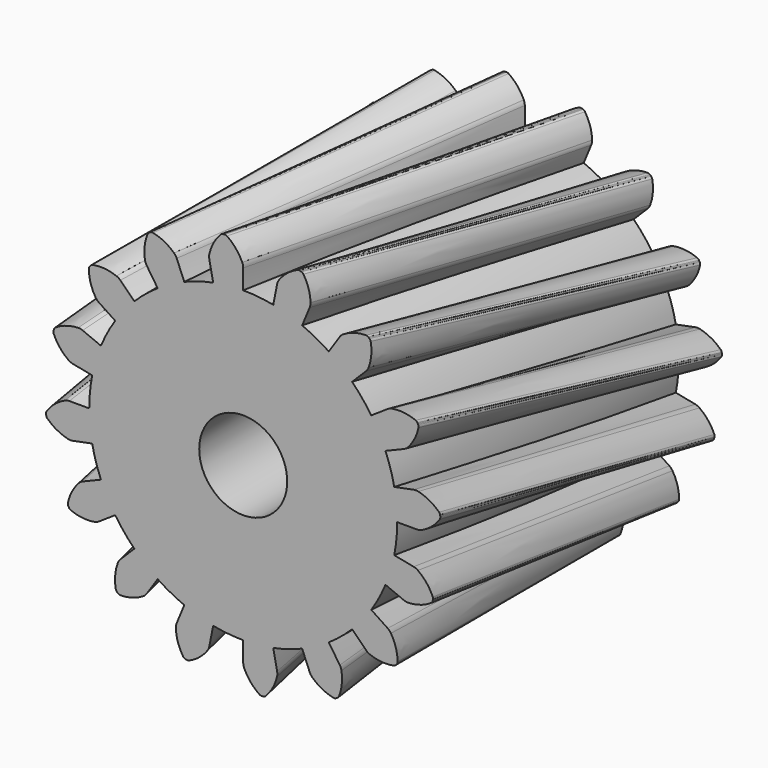
from build123d import *

# Parameters (mm, degrees)
F4_R     = 22.225
F5_DEPTH = 50.8
F6_COUNT = 16
F9_D     = 12.7


with BuildPart() as f3:
    # F0 (on Front) → F3 section 0
    with BuildSketch(Plane.XZ):
        with BuildLine():
            ThreePointArc((-4.3358824068, 21.797952857), (-2.1784309438, 22.1179805503), (0, 22.225))
            Line((0, 22.225), (0, 25.0832488349))
            ThreePointArc((0, 25.0832488349), (-0.0356671724, 25.4178697029), (-0.1410659846, 25.7374543753))
            ThreePointArc((-0.1410659846, 25.7374543753), (-1.0620560581, 27.2018999668), (-2.3441181542, 28.3634249934))
            ThreePointArc((-2.3441181542, 28.3634249934), (-2.5021196775, 28.4354511085), (-2.675148388, 28.4500561742))
            Line((-2.675148388, 28.4500561742), (-2.8009980611, 28.4390105698))
            Line((-2.8009980611, 28.4390105698), (-2.9265844586, 28.4252918828))
            ThreePointArc((-2.9265844586, 28.4252918828), (-3.0934391639, 28.3772112224), (-3.2343531342, 28.2757445009))
            ThreePointArc((-3.2343531342, 28.2757445009), (-4.2651784752, 26.8864199448), (-4.8827728207, 25.2704370147))
            ThreePointArc((-4.8827728207, 25.2704370147), (-4.9237985476, 24.936430784), (-4.8934990924, 24.601281242))
            Line((-4.8934990924, 24.601281242), (-4.3358824068, 21.797952857))
        make_face()
    # F2 (on offset) → F3 section 1
    with BuildSketch(Plane.XZ.offset(50.8)):
        with BuildLine():
            ThreePointArc((-12.3475484289, 18.4794121334), (-10.476792476, 19.6007001001), (-8.5051392843, 20.5332226101))
            Line((-8.5051392843, 20.5332226101), (-9.598943759, 23.1739002075))
            ThreePointArc((-9.598943759, 23.1739002075), (-9.7599497919, 23.4694003426), (-9.9796253566, 23.7243237011))
            ThreePointArc((-9.9796253566, 23.7243237011), (-11.3909283006, 24.724847367), (-13.0198956146, 25.3073326422))
            ThreePointArc((-13.0198956146, 25.3073326422), (-13.193433189, 25.3134115305), (-13.3588799898, 25.2606896309))
            Line((-13.3588799898, 25.2606896309), (-13.4709229572, 25.2023242382))
            Line((-13.4709229572, 25.2023242382), (-13.5816997451, 25.1415899904))
            ThreePointArc((-13.5816997451, 25.1415899904), (-13.7174537202, 25.0333167211), (-13.8088116199, 24.885648252))
            ThreePointArc((-13.8088116199, 24.885648252), (-14.2294985642, 23.2075999509), (-14.1816714451, 21.478283273))
            ThreePointArc((-14.1816714451, 21.478283273), (-14.0917556237, 21.1540018867), (-13.9355064001, 20.8559591841))
            Line((-13.9355064001, 20.8559591841), (-12.3475484289, 18.4794121334))
        make_face()
    loft()

    # F4 (on offset) → F5 (join)
    with BuildSketch(Plane.XZ.offset(50.8)):
        Circle(F4_R)
    extrude(amount=-F5_DEPTH)


with BuildPart() as f6_1:
    # F6: instance of F3
    add(f3.part.rotate(Axis((0, -50.8, 0), (0, -1, 0)), 1 * 360 / F6_COUNT))


with BuildPart() as f6_2:
    # F6: instance of F3
    add(f3.part.rotate(Axis((0, -50.8, 0), (0, -1, 0)), 2 * 360 / F6_COUNT))


with BuildPart() as f6_3:
    # F6: instance of F3
    add(f3.part.rotate(Axis((0, -50.8, 0), (0, -1, 0)), 3 * 360 / F6_COUNT))


with BuildPart() as f6_4:
    # F6: instance of F3
    add(f3.part.rotate(Axis((0, -50.8, 0), (0, -1, 0)), 4 * 360 / F6_COUNT))


with BuildPart() as f6_5:
    # F6: instance of F3
    add(f3.part.rotate(Axis((0, -50.8, 0), (0, -1, 0)), 5 * 360 / F6_COUNT))


with BuildPart() as f6_6:
    # F6: instance of F3
    add(f3.part.rotate(Axis((0, -50.8, 0), (0, -1, 0)), 6 * 360 / F6_COUNT))


with BuildPart() as f6_7:
    # F6: instance of F3
    add(f3.part.rotate(Axis((0, -50.8, 0), (0, -1, 0)), 7 * 360 / F6_COUNT))


with BuildPart() as f6_8:
    # F6: instance of F3
    add(f3.part.rotate(Axis((0, -50.8, 0), (0, -1, 0)), 8 * 360 / F6_COUNT))


with BuildPart() as f6_9:
    # F6: instance of F3
    add(f3.part.rotate(Axis((0, -50.8, 0), (0, -1, 0)), 9 * 360 / F6_COUNT))


with BuildPart() as f6_10:
    # F6: instance of F3
    add(f3.part.rotate(Axis((0, -50.8, 0), (0, -1, 0)), 10 * 360 / F6_COUNT))


with BuildPart() as f6_11:
    # F6: instance of F3
    add(f3.part.rotate(Axis((0, -50.8, 0), (0, -1, 0)), 11 * 360 / F6_COUNT))


with BuildPart() as f6_12:
    # F6: instance of F3
    add(f3.part.rotate(Axis((0, -50.8, 0), (0, -1, 0)), 12 * 360 / F6_COUNT))


with BuildPart() as f6_13:
    # F6: instance of F3
    add(f3.part.rotate(Axis((0, -50.8, 0), (0, -1, 0)), 13 * 360 / F6_COUNT))


with BuildPart() as f6_14:
    # F6: instance of F3
    add(f3.part.rotate(Axis((0, -50.8, 0), (0, -1, 0)), 14 * 360 / F6_COUNT))


with BuildPart() as f6_15:
    # F6: instance of F3
    add(f3.part.rotate(Axis((0, -50.8, 0), (0, -1, 0)), 15 * 360 / F6_COUNT))


with BuildPart() as f6_8_1:
    add(f6_8.part)

    # F7: union F6_9, F6_10, F6_11, F6_12, F6_13, F6_14, F6_15, F3, F6_1, F6_2, F6_3, F6_4, F6_5, F6_6, F6_7
    add(f6_9.part)
    add(f6_10.part)
    add(f6_11.part)
    add(f6_12.part)
    add(f6_13.part)
    add(f6_14.part)
    add(f6_15.part)
    add(f3.part)
    add(f6_1.part)
    add(f6_2.part)
    add(f6_3.part)
    add(f6_4.part)
    add(f6_5.part)
    add(f6_6.part)
    add(f6_7.part)

    # F9 (through all)
    with Locations(Plane.XZ.offset(50.8)):
        with Locations((0, 0)):
            Hole(F9_D / 2)


solid = f6_8_1.part
